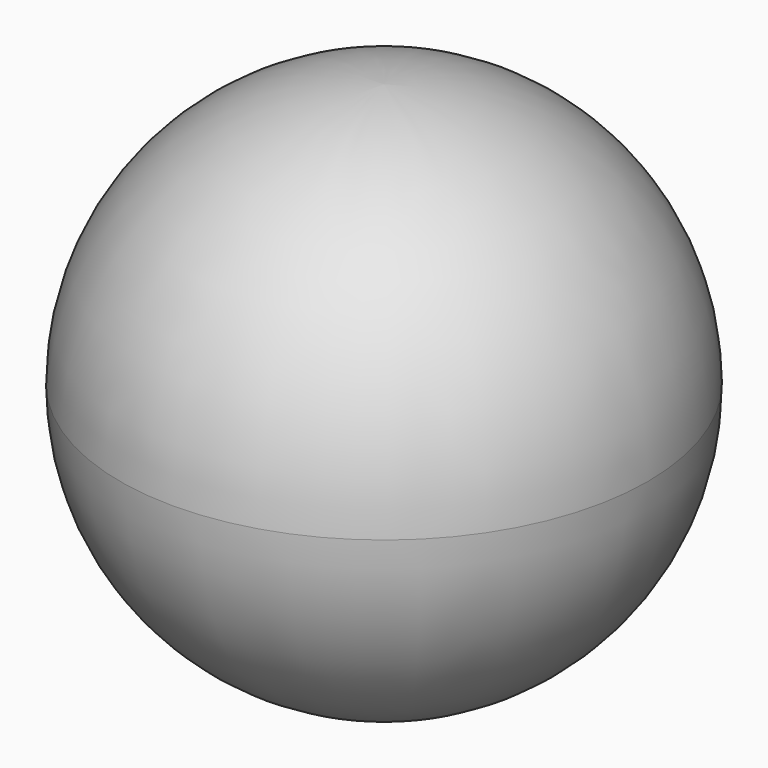
from build123d import *

# Parameters (mm, degrees)
F0_R          = 15.5
F1_DEPTH      = 15.5
F1_DEPTH_BACK = 15.5
F2_R          = 15.49999


# Not quite as in the source:
# - a fillet or chamfer is up to 0.001 mm smaller than in the source, because OpenCascade refuses the exact size


with BuildPart() as f1:
    # F0 (on Top) → F1 (new body, two sides)
    with BuildSketch(Plane.XY) as f1_sk:
        Circle(F0_R)
    extrude(amount=F1_DEPTH)
    extrude(f1_sk.sketch, amount=-F1_DEPTH_BACK)

    # F2 (radius 15.5 in the source; OpenCascade refuses exactly that, so slightly less here)
    f2_edges = [f1.edges().sort_by_distance(p)[0] for p in [
        (-15.5, 0, 15.5),
        (-15.5, 0, -15.5),
    ]]
    fillet(f2_edges, radius=F2_R)


solid = f1.part
